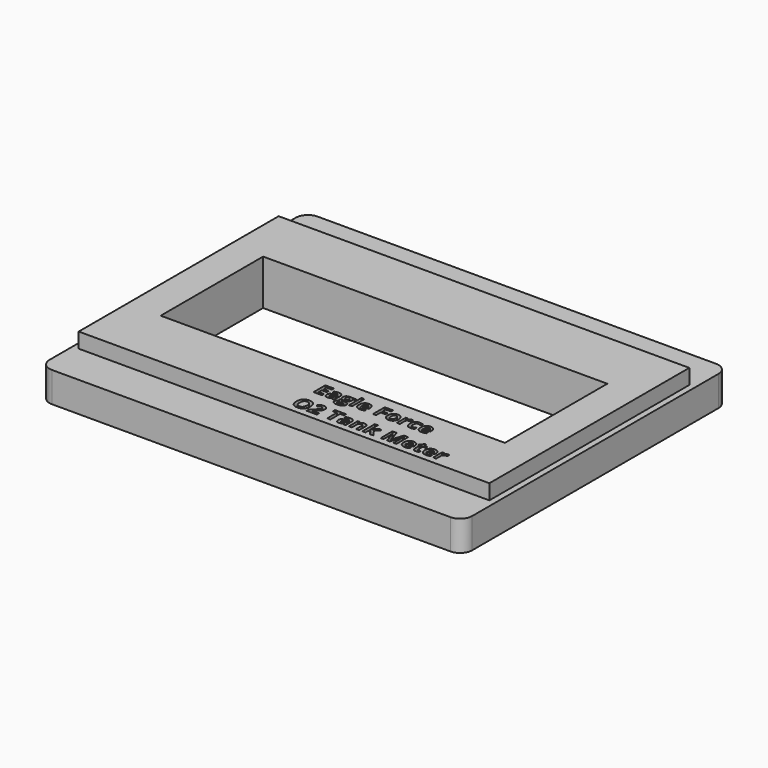
from build123d import *

# Parameters (mm, degrees)
F0_W          = 88.9
F0_H          = 69.85
F1_DEPTH      = 6.35
F6_R          = 2.54
F7_W          = 86.36
F7_H          = 52.5526
F8_DEPTH      = 3.175
F5_W          = 72.39
F5_H          = 26.924
F9_DEPTH      = 25.4
F9_DEPTH_BACK = 3.176
F10_TEXT_SIZE = 4.331386659
F11_DEPTH     = 6.35


# Not quite as in the source:
# - Text() gives the source's letters only with a copy of the font that has no kerning and outlines rounded to 1/6400 em; it was checked with that copy


with BuildPart() as f1:
    # F0 (on Top) → F1 (new body)
    with BuildSketch(Plane.XY):
        Rectangle(F0_W, F0_H)
    extrude(amount=F1_DEPTH)

    # F3: F1 across plane


with BuildPart() as f1_1:
    add(f1.part)
    add(f1.part.mirror(Plane.XZ))

    # F4: F1 across plane


with BuildPart() as f1_2:
    add(f1_1.part)
    add(f1_1.part.mirror(Plane.YZ))

    # F6
    f6_edges = [f1_2.edges().sort_by_distance(p)[0] for p in [
        (44.45, 34.925, 3.175),
        (-44.45, 34.925, 3.175),
        (-44.45, -34.925, 3.175),
        (44.45, -34.925, 3.175),
    ]]
    fillet(f6_edges, radius=F6_R)

    # F7 (on face) → F8 (join)
    with BuildSketch(Plane.XY.offset(6.35)):
        Rectangle(F7_W, F7_H)
    extrude(amount=F8_DEPTH)

    # F5 (on face) → F9 (cut, two sides)
    with BuildSketch(Plane.XY.offset(6.35)) as f9_sk:
        Rectangle(F5_W, F5_H)
    extrude(amount=-F9_DEPTH, mode=Mode.SUBTRACT)
    extrude(f9_sk.sketch, amount=F9_DEPTH_BACK, mode=Mode.SUBTRACT)

    # F10 (on face) → F11 (cut)
    with BuildSketch(Plane.XY.offset(6.35)):
        with Locations((0, -19.0012529492)):
            Text('Eagle Force', F10_TEXT_SIZE, font='Open Sans', font_style=FontStyle.BOLD, text_align=(TextAlign.LEFT, TextAlign.BOTTOM))
        with Locations((0, -24.8919388055)):
            Text('O2 Tank Meter', F10_TEXT_SIZE, font='Open Sans', font_style=FontStyle.BOLD, text_align=(TextAlign.LEFT, TextAlign.BOTTOM))
        with Locations((0, -30.7826246617)):
            Text('V1.0', F10_TEXT_SIZE, font='Open Sans', font_style=FontStyle.BOLD, text_align=(TextAlign.LEFT, TextAlign.BOTTOM))
    extrude(amount=F11_DEPTH, mode=Mode.SUBTRACT)


solid = f1_2.part
